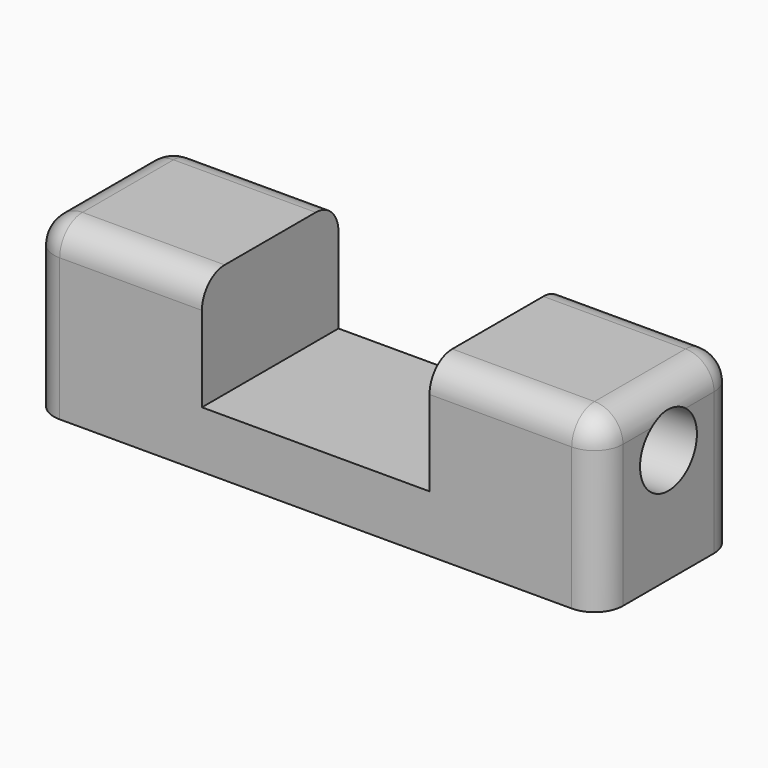
from build123d import *

# Parameters (mm, degrees)
F1_DEPTH     = 60
F2_R         = 12.5
F3_DEPTH     = 70
F4_T1_DEPTH  = 75
F4_T3_DEPTH  = 40
F4_T5_DEPTH  = 75
F4_T7_DEPTH  = 75
F4_S11_W     = 10
F4_S11_H     = 10
F4_T12_DEPTH = 10
F4_S17_W     = 10
F4_S17_H     = 10
F4_T18_DEPTH = 10
F4_S23_W     = 10
F4_S23_H     = 10
F4_T24_DEPTH = 10
F4_S29_W     = 10
F4_S29_H     = 10
F4_T30_DEPTH = 10


# Not quite as in the source:
# - a fillet or chamfer that OpenCascade refuses, or shapes differently, is made with other operations: its cross-section is extruded or revolved along the edge and cut away or added


with BuildPart() as f1:
    # F0 (on Front) → F1 (new body)
    with BuildSketch(Plane.XZ):
        Polygon((0, 60), (0, 0), (200, 0), (200, 60), (140, 60), (140, 20), (60, 20), (60, 60), align=None)
    extrude(amount=F1_DEPTH)

    # F2 (on face) → F3 (cut)
    with BuildSketch(Plane.YZ.offset(200)):
        with Locations((-30, 40)):
            Circle(F2_R)
    extrude(amount=-F3_DEPTH, mode=Mode.SUBTRACT)

    # F4: fillet of radius 10 on 10 edges, made by hand

    # F4_s2 → F4_t1 (cut)
    with BuildSketch(Plane.XY.offset(-25)):
        with BuildLine():
            ThreePointArc((0, -50), (2.9289321881, -57.0710678119), (10, -60))
            Line((10, -60), (0, -60))
            Line((0, -60), (0, -50))
        make_face()
        with BuildLine():
            ThreePointArc((0, -10), (2.9289321881, -2.9289321881), (10, 0))
            Line((10, 0), (0, 0))
            Line((0, 0), (0, -10))
        make_face()
        with BuildLine():
            ThreePointArc((190, -60), (197.0710678119, -57.0710678119), (200, -50))
            Line((200, -50), (200, -60))
            Line((200, -60), (190, -60))
        make_face()
        with BuildLine():
            ThreePointArc((190, 0), (197.0710678119, -2.9289321881), (200, -10))
            Line((200, -10), (200, 0))
            Line((200, 0), (190, 0))
        make_face()
    extrude(amount=F4_T1_DEPTH, mode=Mode.SUBTRACT)

    # F4_s4 → F4_t3 (cut)
    with BuildSketch(Plane.XZ.offset(10)):
        with BuildLine():
            ThreePointArc((0, 50), (2.9289321881, 57.0710678119), (10, 60))
            Line((10, 60), (0, 60))
            Line((0, 60), (0, 50))
        make_face()
        with BuildLine():
            ThreePointArc((200, 50), (197.0710678119, 57.0710678119), (190, 60))
            Line((190, 60), (200, 60))
            Line((200, 60), (200, 50))
        make_face()
    extrude(amount=F4_T3_DEPTH, mode=Mode.SUBTRACT)

    # F4_s6 → F4_t5 (cut)
    with BuildSketch(Plane.YZ.offset(10)):
        with BuildLine():
            ThreePointArc((-10, 60), (-2.9289321881, 57.0710678119), (0, 50))
            Line((0, 50), (0, 60))
            Line((0, 60), (-10, 60))
        make_face()
        with BuildLine():
            ThreePointArc((-50, 60), (-57.0710678119, 57.0710678119), (-60, 50))
            Line((-60, 50), (-60, 60))
            Line((-60, 60), (-50, 60))
        make_face()
    extrude(amount=F4_T5_DEPTH, mode=Mode.SUBTRACT)

    # F4_s8 → F4_t7 (cut)
    with BuildSketch(Plane.YZ.offset(115)):
        with BuildLine():
            ThreePointArc((-60, 50), (-57.0710678119, 57.0710678119), (-50, 60))
            Line((-50, 60), (-60, 60))
            Line((-60, 60), (-60, 50))
        make_face()
        with BuildLine():
            ThreePointArc((0, 50), (-2.9289321881, 57.0710678119), (-10, 60))
            Line((-10, 60), (0, 60))
            Line((0, 60), (0, 50))
        make_face()
    extrude(amount=F4_T7_DEPTH, mode=Mode.SUBTRACT)


with BuildPart() as f4_tool10:
    # F4_s11 → F4_t12 (new body)
    with BuildSketch(Plane.YZ.offset(10)):
        with Locations((-55, 55)):
            Rectangle(F4_S11_W, F4_S11_H)
    extrude(amount=-F4_T12_DEPTH)

    # F4_s13 → F4_t14 (revolve, cut)
    with BuildSketch(Plane(origin=(10, -50, 50), x_dir=(0, 0.7071067812, -0.7071067812), z_dir=(0, 0.7071067812, 0.7071067812))):
        with BuildLine():
            ThreePointArc((0, -10), (10, 0), (0, 10))
            Line((0, 10), (0, -10))
        make_face()
    revolve(axis=Axis((10, -50, 50), (-1, 0, 0)), mode=Mode.SUBTRACT)


with BuildPart() as f1_1:
    add(f1.part)

    # F4_t9: cut F4_tool10
    add(f4_tool10.part, mode=Mode.SUBTRACT)


with BuildPart() as f4_tool16:
    # F4_s17 → F4_t18 (new body)
    with BuildSketch(Plane.YZ.offset(10)):
        with Locations((-5, 55)):
            Rectangle(F4_S17_W, F4_S17_H)
    extrude(amount=-F4_T18_DEPTH)

    # F4_s19 → F4_t20 (revolve, cut)
    with BuildSketch(Plane(origin=(10, -10, 50), x_dir=(0, -0.7071067812, -0.7071067812), z_dir=(0, 0.7071067812, -0.7071067812))):
        with BuildLine():
            ThreePointArc((0, -10), (10, 0), (0, 10))
            Line((0, 10), (0, -10))
        make_face()
    revolve(axis=Axis((10, -10, 50), (-1, 0, 0)), mode=Mode.SUBTRACT)


with BuildPart() as f1_2:
    add(f1_1.part)

    # F4_t15: cut F4_tool16
    add(f4_tool16.part, mode=Mode.SUBTRACT)


with BuildPart() as f4_tool22:
    # F4_s23 → F4_t24 (new body)
    with BuildSketch(Plane.XZ.offset(50)):
        with Locations((195, 55)):
            Rectangle(F4_S23_W, F4_S23_H)
    extrude(amount=F4_T24_DEPTH)

    # F4_s25 → F4_t26 (revolve, cut)
    with BuildSketch(Plane(origin=(190, -50, 50), x_dir=(-0.7071067812, 0, -0.7071067812), z_dir=(-0.7071067812, 0, 0.7071067812))):
        with BuildLine():
            ThreePointArc((0, -10), (10, 0), (0, 10))
            Line((0, 10), (0, -10))
        make_face()
    revolve(axis=Axis((190, -50, 50), (0, -1, 0)), mode=Mode.SUBTRACT)


with BuildPart() as f1_3:
    add(f1_2.part)

    # F4_t21: cut F4_tool22
    add(f4_tool22.part, mode=Mode.SUBTRACT)


with BuildPart() as f4_tool28:
    # F4_s29 → F4_t30 (new body)
    with BuildSketch(Plane.XZ.offset(10)):
        with Locations((195, 55)):
            Rectangle(F4_S29_W, F4_S29_H)
    extrude(amount=-F4_T30_DEPTH)

    # F4_s31 → F4_t32 (revolve, cut)
    with BuildSketch(Plane(origin=(190, -10, 50), x_dir=(-0.7071067812, 0, -0.7071067812), z_dir=(0.7071067812, 0, -0.7071067812))):
        with BuildLine():
            ThreePointArc((0, -10), (10, 0), (0, 10))
            Line((0, 10), (0, -10))
        make_face()
    revolve(axis=Axis((190, -10, 50), (0, 1, 0)), mode=Mode.SUBTRACT)


with BuildPart() as f1_4:
    add(f1_3.part)

    # F4_t27: cut F4_tool28
    add(f4_tool28.part, mode=Mode.SUBTRACT)


solid = f1_4.part
